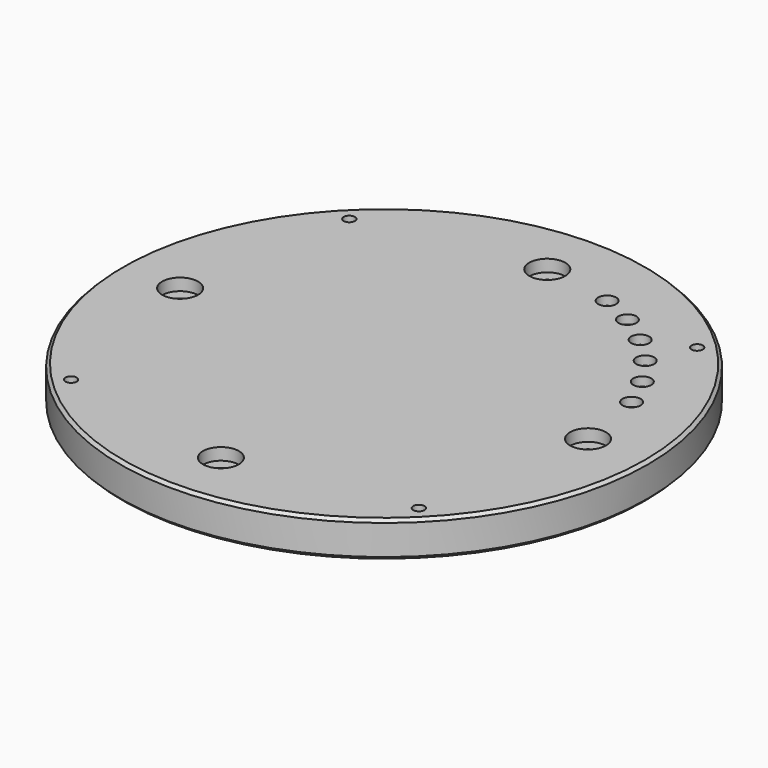
from build123d import *

# Parameters (mm, degrees)
F2_R      = 139.7
F3_DEPTH  = 19.05
F4_SIZE   = 1.5875
F5_R      = 0.79375
F6_DEPTH  = 19.051
F7_R      = 2.9765625
F7_R_2    = 0.79375
F8_DEPTH  = 19.051
F9_R      = 2.9765625
F10_DEPTH = 19.051
F11_R     = 9.525
F11_R_2   = 2.9765625
F12_DEPTH = 6.35
F13_R     = 3.175
F14_DEPTH = 19.051
F15_R     = 1.1938
F16_DEPTH = 12.7
F17_R     = 7.9375
F17_R_2   = 3.175
F17_R_3   = 1.1938
F18_DEPTH = 10.16
F19_R     = 4.7625
F19_R_2   = 3.175
F20_DEPTH = 4.7752


# Not quite as in the source:
# - a variable given as a bare number and used for a length is read in inches; the dataset says mm whatever the document's units were


with BuildPart() as f3:
    # F2 (on Top) → F3 (new body)
    with BuildSketch(Plane.XY):
        Circle(F2_R)
    extrude(amount=F3_DEPTH)

    # F4
    f4_edges = [f3.edges().sort_by_distance(p)[0] for p in [
        (-139.7, 0, 19.05),
        (-139.7, 0, 0),
    ]]
    chamfer(f4_edges, length=F4_SIZE)

    # F5 (on face) → F6 (cut, through all)
    with BuildSketch(Plane.XY.offset(19.05)):
        with Locations((-92.047625241, 92.047625241)):
            Circle(F5_R)
        with Locations((92.047625241, 92.047625241)):
            Circle(F5_R)
        with Locations((92.047625241, -92.047625241)):
            Circle(F5_R)
        with Locations((-92.047625241, -92.047625241)):
            Circle(F5_R)
    extrude(amount=-F6_DEPTH, mode=Mode.SUBTRACT)

    # F7 (on face) → F8 (cut, through all)
    with BuildSketch(Plane.XY.offset(19.05)):
        with Locations((-92.047625241, 92.047625241)):
            Circle(F7_R)
        with Locations((-92.047625241, 92.047625241)):
            Circle(F7_R_2, mode=Mode.SUBTRACT)
        with Locations((92.047625241, 92.047625241)):
            Circle(F7_R)
        with Locations((92.047625241, 92.047625241)):
            Circle(F7_R_2, mode=Mode.SUBTRACT)
        with Locations((-92.047625241, -92.047625241)):
            Circle(F7_R)
        with Locations((-92.047625241, -92.047625241)):
            Circle(F7_R_2, mode=Mode.SUBTRACT)
        with Locations((92.047625241, -92.047625241)):
            Circle(F7_R)
        with Locations((92.047625241, -92.047625241)):
            Circle(F7_R_2, mode=Mode.SUBTRACT)
    extrude(amount=-F8_DEPTH, mode=Mode.SUBTRACT)

    # F9 (on face) → F10 (cut, through all)
    with BuildSketch(Plane.XY.offset(19.05)):
        with Locations((0, 107.95)):
            Circle(F9_R)
        with Locations((107.95, 0)):
            Circle(F9_R)
        with Locations((0, -107.95)):
            Circle(F9_R)
        with Locations((-107.95, 0)):
            Circle(F9_R)
    extrude(amount=-F10_DEPTH, mode=Mode.SUBTRACT)

    # F11 (on face) → F12 (cut)
    with BuildSketch(Plane.XY.offset(19.05)):
        with Locations((0, 107.95)):
            Circle(F11_R)
        with Locations((0, 107.95)):
            Circle(F11_R_2, mode=Mode.SUBTRACT)
        with Locations((107.95, 0)):
            Circle(F11_R)
        with Locations((107.95, 0)):
            Circle(F11_R_2, mode=Mode.SUBTRACT)
        with Locations((0, -107.95)):
            Circle(F11_R)
        with Locations((0, -107.95)):
            Circle(F11_R_2, mode=Mode.SUBTRACT)
        with Locations((-107.95, 0)):
            Circle(F11_R)
        with Locations((-107.95, 0)):
            Circle(F11_R_2, mode=Mode.SUBTRACT)
    extrude(amount=-F12_DEPTH, mode=Mode.SUBTRACT)

    # F13 (on face) → F14 (cut, through all)
    with BuildSketch(Plane.XY.offset(19.05)):
        with Locations((36.921074472, 101.4398184138)):
            Circle(F13_R)
        with Locations((53.975, 93.4874423385)):
            Circle(F13_R)
        with Locations((69.3889224657, 82.6944976347)):
            Circle(F13_R)
        with Locations((82.6944976347, 69.3889224657)):
            Circle(F13_R)
        with Locations((93.4874423385, 53.975)):
            Circle(F13_R)
        with Locations((101.4398184138, 36.921074472)):
            Circle(F13_R)
    extrude(amount=-F14_DEPTH, mode=Mode.SUBTRACT)

    # F15 (on face) → F16 (cut)
    with BuildSketch(Plane(origin=(0, 0, 0), x_dir=(1, 0, 0), z_dir=(0, 0, -1))):
        with Locations((50.927, -88.2081514771)):
            Circle(F15_R)
        with Locations((65.470489197, -78.0246907094)):
            Circle(F15_R)
        with Locations((78.0246907094, -65.470489197)):
            Circle(F15_R)
        with Locations((88.2081514771, -50.927)):
            Circle(F15_R)
        with Locations((95.7114521975, -34.8361196783)):
            Circle(F15_R)
        with Locations((34.8361196783, -95.7114521975)):
            Circle(F15_R)
    extrude(amount=-F16_DEPTH, mode=Mode.SUBTRACT)

    # F17 (on face) → F18 (cut)
    with BuildSketch(Plane(origin=(0, 0, 0), x_dir=(1, 0, 0), z_dir=(0, 0, -1))):
        with Locations((36.921074472, -101.4398184138)):
            Circle(F17_R)
        with Locations((36.921074472, -101.4398184138)):
            Circle(F17_R_2, mode=Mode.SUBTRACT)
        with Locations((34.8361196783, -95.7114521975)):
            Circle(F17_R_3, mode=Mode.SUBTRACT)
        with Locations((53.975, -93.4874423385)):
            Circle(F17_R)
        with Locations((50.927, -88.2081514771)):
            Circle(F17_R_3, mode=Mode.SUBTRACT)
        with Locations((53.975, -93.4874423385)):
            Circle(F17_R_2, mode=Mode.SUBTRACT)
        with Locations((69.3889224657, -82.6944976347)):
            Circle(F17_R)
        with Locations((65.470489197, -78.0246907094)):
            Circle(F17_R_3, mode=Mode.SUBTRACT)
        with Locations((69.3889224657, -82.6944976347)):
            Circle(F17_R_2, mode=Mode.SUBTRACT)
        with Locations((82.6944976347, -69.3889224657)):
            Circle(F17_R)
        with Locations((82.6944976347, -69.3889224657)):
            Circle(F17_R_2, mode=Mode.SUBTRACT)
        with Locations((78.0246907094, -65.470489197)):
            Circle(F17_R_3, mode=Mode.SUBTRACT)
        with Locations((93.4874423385, -53.975)):
            Circle(F17_R)
        with Locations((93.4874423385, -53.975)):
            Circle(F17_R_2, mode=Mode.SUBTRACT)
        with Locations((88.2081514771, -50.927)):
            Circle(F17_R_3, mode=Mode.SUBTRACT)
        with Locations((101.4398184138, -36.921074472)):
            Circle(F17_R)
        with Locations((95.7114521975, -34.8361196783)):
            Circle(F17_R_3, mode=Mode.SUBTRACT)
        with Locations((101.4398184138, -36.921074472)):
            Circle(F17_R_2, mode=Mode.SUBTRACT)
    extrude(amount=-F18_DEPTH, mode=Mode.SUBTRACT)

    # F19 (on face) → F20 (cut)
    with BuildSketch(Plane.XY.offset(19.05)):
        with Locations((36.921074472, 101.4398184138)):
            Circle(F19_R)
        with Locations((36.921074472, 101.4398184138)):
            Circle(F19_R_2, mode=Mode.SUBTRACT)
        with Locations((53.975, 93.4874423385)):
            Circle(F19_R)
        with Locations((53.975, 93.4874423385)):
            Circle(F19_R_2, mode=Mode.SUBTRACT)
        with Locations((69.3889224657, 82.6944976347)):
            Circle(F19_R)
        with Locations((69.3889224657, 82.6944976347)):
            Circle(F19_R_2, mode=Mode.SUBTRACT)
        with Locations((82.6944976347, 69.3889224657)):
            Circle(F19_R)
        with Locations((82.6944976347, 69.3889224657)):
            Circle(F19_R_2, mode=Mode.SUBTRACT)
        with Locations((93.4874423385, 53.975)):
            Circle(F19_R)
        with Locations((93.4874423385, 53.975)):
            Circle(F19_R_2, mode=Mode.SUBTRACT)
        with Locations((101.4398184138, 36.921074472)):
            Circle(F19_R)
        with Locations((101.4398184138, 36.921074472)):
            Circle(F19_R_2, mode=Mode.SUBTRACT)
    extrude(amount=-F20_DEPTH, mode=Mode.SUBTRACT)


solid = f3.part
